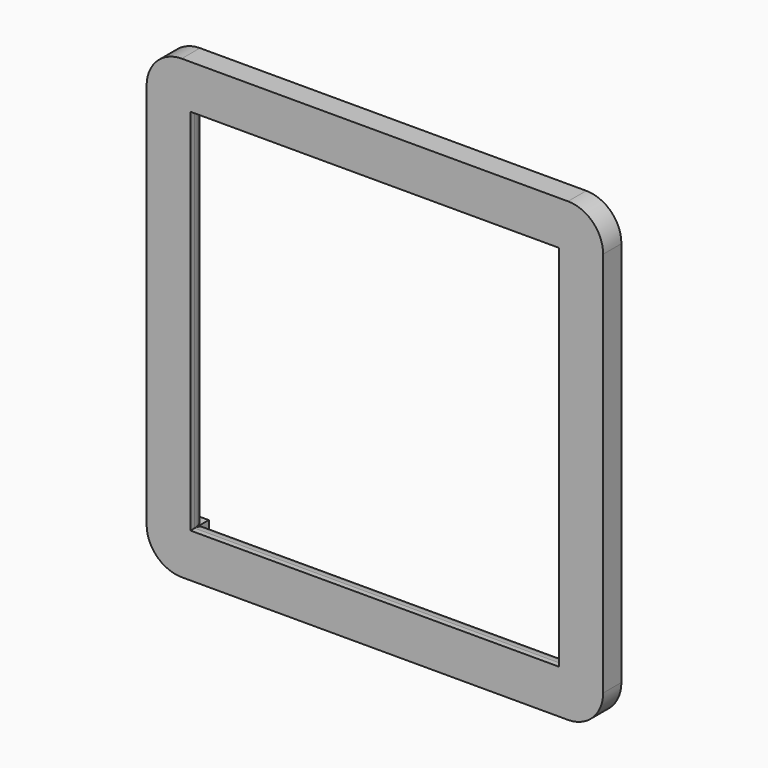
from build123d import *

# Parameters (mm, degrees)
F0_W     = 66.04
F0_H     = 66.04
F0_W_2   = 53.34
F0_H_2   = 53.34
F1_DEPTH = 3.302
F2_R     = 5.08
F3_W     = 53.34
F3_H     = 3.81
F3_W_2   = 3.81
F3_H_2   = 53.34
F4_DEPTH = 2.54
F6_W     = 53.34
F6_H     = 3.81
F9_DEPTH = 2.54
F5_W     = 3.81
F5_H     = 53.34
F8_W     = 53.34
F8_H     = 3.81
F7_W     = 3.81
F7_H     = 53.34
F10_R    = 2.53999
F10_2_R  = 2.53999
F10_3_R  = 2.53999
F10_4_R  = 2.53999


# Not quite as in the source:
# - a fillet or chamfer is up to 0.001 mm smaller than in the source, because OpenCascade refuses the exact size


with BuildPart() as f1:
    # F0 (on Front) → F1 (new body)
    with BuildSketch(Plane.XZ):
        with Locations((-340.0468912915, -298.0797665718)):
            Rectangle(F0_W, F0_H)
        with Locations((-340.0468912915, -298.0797665718)):
            Rectangle(F0_W_2, F0_H_2, mode=Mode.SUBTRACT)
    extrude(amount=F1_DEPTH)

    # F2
    f2_edges = [f1.edges().sort_by_distance(p)[0] for p in [
        (-307.026891, -1.651, -331.099767),
        (-373.066891, -1.651, -331.099767),
        (-373.066891, -1.651, -265.059767),
        (-307.026891, -1.651, -265.059767),
    ]]
    fillet(f2_edges, radius=F2_R)

    # F3 (on face) → F4 (cut)
    with BuildSketch(Plane(origin=(0, 0, 0), x_dir=(-1, 0, 0), z_dir=(0, 1, 0))):
        with Locations((340.0468912915, -326.6547665718)):
            Rectangle(F3_W, F3_H)
        with Locations((368.6218912915, -298.0797665718)):
            Rectangle(F3_W_2, F3_H_2)
        with Locations((340.0468912915, -269.5047665718)):
            Rectangle(F3_W, F3_H)
        with Locations((311.4718912915, -298.0797665718)):
            Rectangle(F3_W_2, F3_H_2)
    extrude(amount=-F4_DEPTH, mode=Mode.SUBTRACT)


with BuildPart() as f9:
    # F6 (on face) → F9 (new body)
    with BuildSketch(Plane(origin=(0, -2.54, 0), x_dir=(-1, 0, 0), z_dir=(0, 1, 0))):
        with Locations((340.0468912915, -326.6547665718)):
            Rectangle(F6_W, F6_H)
    extrude(amount=F9_DEPTH)

    # F10#2 (radius 2.54 in the source; OpenCascade refuses exactly that, so slightly less here)
    f10_2_edges = [f9.edges().sort_by_distance(p)[0] for p in [
        (-340.046891, 0, -324.749767),
    ]]
    fillet(f10_2_edges, radius=F10_2_R)


with BuildPart() as f9b:
    # F5 (on face) → F9, piece 2 (new body)
    with BuildSketch(Plane(origin=(0, -2.54, 0), x_dir=(-1, 0, 0), z_dir=(0, 1, 0))):
        with Locations((311.4718912915, -298.0797665718)):
            Rectangle(F5_W, F5_H)
    extrude(amount=F9_DEPTH)

    # F10 (radius 2.54 in the source; OpenCascade refuses exactly that, so slightly less here)
    f10_edges = [f9b.edges().sort_by_distance(p)[0] for p in [
        (-313.376891, 0, -298.079767),
    ]]
    fillet(f10_edges, radius=F10_R)


with BuildPart() as f9c:
    # F8 (on face) → F9, piece 3 (new body)
    with BuildSketch(Plane(origin=(0, -2.54, 0), x_dir=(-1, 0, 0), z_dir=(0, 1, 0))):
        with Locations((340.0468912915, -269.5047665718)):
            Rectangle(F8_W, F8_H)
    extrude(amount=F9_DEPTH)

    # F10#4 (radius 2.54 in the source; OpenCascade refuses exactly that, so slightly less here)
    f10_4_edges = [f9c.edges().sort_by_distance(p)[0] for p in [
        (-340.046891, 0, -271.409767),
    ]]
    fillet(f10_4_edges, radius=F10_4_R)


with BuildPart() as f9d:
    # F7 (on face) → F9, piece 4 (new body)
    with BuildSketch(Plane(origin=(0, -2.54, 0), x_dir=(-1, 0, 0), z_dir=(0, 1, 0))):
        with Locations((368.6218912915, -298.0797665718)):
            Rectangle(F7_W, F7_H)
    extrude(amount=F9_DEPTH)

    # F10#3 (radius 2.54 in the source; OpenCascade refuses exactly that, so slightly less here)
    f10_3_edges = [f9d.edges().sort_by_distance(p)[0] for p in [
        (-366.716891, 0, -298.079767),
    ]]
    fillet(f10_3_edges, radius=F10_3_R)


solid = Compound([f1.part, f9.part, f9b.part, f9c.part, f9d.part])
